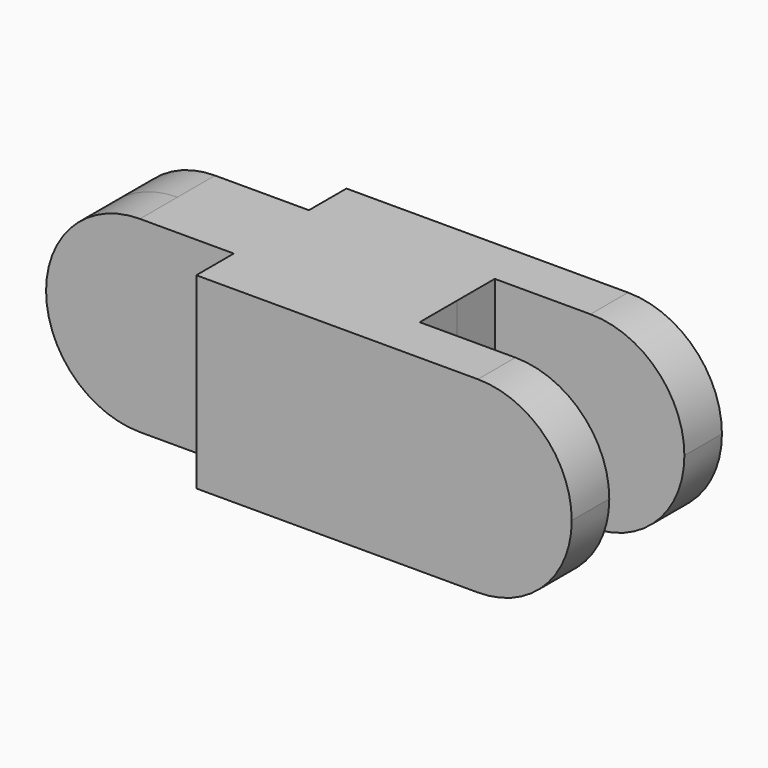
from build123d import *

# Parameters (mm, degrees)
F1_DEPTH = 3.175
F2_W     = 25.4
F2_H     = 12.7
F3_DEPTH = 3.175
F4_R     = 6.34999
F5_W     = 12.954
F5_H     = 3.175
F6_DEPTH = 25.4


# Not quite as in the source:
# - a fillet or chamfer is up to 0.001 mm smaller than in the source, because OpenCascade refuses the exact size


with BuildPart() as f1:
    # F0 (on Front) → F1 (new body)
    with BuildSketch(Plane.XZ):
        with BuildLine():
            ThreePointArc((0, 6.35), (1.8598719395, 1.8598719395), (6.35, 0))
            Line((6.35, 0), (38.1, 0))
            Line((38.1, 0), (38.1, 12.7))
            Line((38.1, 12.7), (6.35, 12.7))
            ThreePointArc((6.35, 12.7), (1.8598719395, 10.8401280605), (0, 6.35))
        make_face()
    extrude(amount=F1_DEPTH)

    # F2 (on face) → F3 (join)
    with BuildSketch(Plane.XZ.offset(3.175)):
        with Locations((25.4, 6.35)):
            Rectangle(F2_W, F2_H)
    extrude(amount=F3_DEPTH)

    # F4 (radius 6.35 in the source; OpenCascade refuses exactly that, so slightly less here)
    f4_edges = [f1.edges().sort_by_distance(p)[0] for p in [
        (38.1, -3.175, 12.7),
        (38.1, -3.175, 0),
    ]]
    fillet(f4_edges, radius=F4_R)

    # F5 (on face) → F6 (cut)
    with BuildSketch(Plane.XY.offset(12.7)):
        with Locations((31.75, -1.5875)):
            Rectangle(F5_W, F5_H)
    extrude(amount=-F6_DEPTH, mode=Mode.SUBTRACT)

    # F7: F1 across face


with BuildPart() as f1_1:
    add(f1.part)
    add(f1.part.mirror(Plane(origin=(13.2758554346, 0, 6.35), x_dir=(1, 0, 0), z_dir=(0, 1, 0))))


solid = f1_1.part
